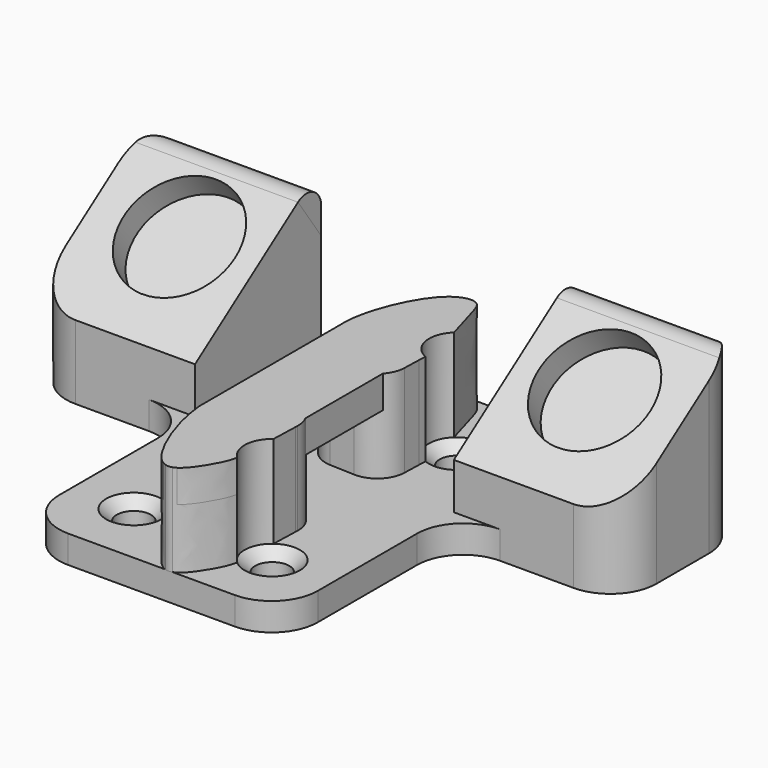
from build123d import *

# Parameters (mm, degrees)
F0_W            = 28.0605573207
F0_H            = 17.1019586477
F1_DEPTH        = 3
F3_DEPTH        = 32
F3_DEPTH_BACK   = 32
F4_DEPTH        = 25
F5_W            = 28.0605573207
F5_H            = 17.0454510609
F5_H_2          = 8.3564384666
F6_REACH        = 49.2047839512
F5_R            = 6.05
F7_DEPTH        = 3
F9_DEPTH        = 10
F10_D           = 3.7
F10_CSINK_D     = 6
F10_CSINK_ANGLE = 90
F12_DEPTH       = 25
F13_DEPTH       = 25
F14_DEPTH       = 5


# Not quite as in the source:
# - a feature names something its author has since deleted; it is built from what else it names


with BuildPart() as f1:
    # F0 (on Top) → F1 (new body)
    with BuildSketch(Plane.XY):
        with BuildLine():
            Line((-19.0302786604, -1.7378998397), (-14.0302786604, -1.7378998397))
            Line((-14.0302786604, -1.7378998397), (-14.0302786604, 15.3640588081))
            Line((-14.0302786604, 15.3640588081), (-27, 15.3640588081))
            ThreePointArc((-27, 15.3640588081), (-30.5355339059, 13.899592714), (-32, 10.3640588081))
            Line((-32, 10.3640588081), (-32, 3.2621001603))
            ThreePointArc((-32, 3.2621001603), (-30.5355339059, -0.2734337456), (-27, -1.7378998397))
            Line((-27, -1.7378998397), (-20.8602603525, -1.7378998397))
            Line((-20.8602603525, -1.7378998397), (-19.0302786604, -1.7378998397))
        make_face()
        with BuildLine():
            ThreePointArc((-14.0302786604, -20.1735929717), (-12.5658125663, -23.7091268776), (-9.0302786604, -25.1735929717))
            Line((-9.0302786604, -25.1735929717), (9.0302786604, -25.1735929717))
            ThreePointArc((9.0302786604, -25.1735929717), (12.5658125663, -23.7091268776), (14.0302786604, -20.1735929717))
            Line((14.0302786604, -20.1735929717), (14.0302786604, -6.7378998397))
            Line((14.0302786604, -6.7378998397), (14.0302786604, -1.7378998397))
            Line((14.0302786604, -1.7378998397), (-14.0302786604, -1.7378998397))
            Line((-14.0302786604, -1.7378998397), (-14.0302786604, -6.7378998397))
            Line((-14.0302786604, -6.7378998397), (-14.0302786604, -20.1735929717))
        make_face()
        with BuildLine():
            Line((14.0302786604, 15.3640588081), (14.0302786604, -1.7378998397))
            Line((14.0302786604, -1.7378998397), (19.0302786604, -1.7378998397))
            Line((19.0302786604, -1.7378998397), (21.6872710735, -1.7378998397))
            Line((21.6872710735, -1.7378998397), (27, -1.7378998397))
            ThreePointArc((27, -1.7378998397), (30.5355339059, -0.2734337456), (32, 3.2621001603))
            Line((32, 3.2621001603), (32, 10.3640588081))
            ThreePointArc((32, 10.3640588081), (30.5355339059, 13.899592714), (27, 15.3640588081))
            Line((27, 15.3640588081), (14.0302786604, 15.3640588081))
        make_face()
        with Locations((0, 6.8130794842)):
            Rectangle(F0_W, F0_H)
        with BuildLine():
            ThreePointArc((-19.0302786604, -1.7378998397), (-15.4947447544, -3.2023659338), (-14.0302786604, -6.7378998397))
            Line((-14.0302786604, -6.7378998397), (-14.0302786604, -1.7378998397))
            Line((-14.0302786604, -1.7378998397), (-19.0302786604, -1.7378998397))
        make_face()
        with BuildLine():
            Line((14.0302786604, -1.7378998397), (14.0302786604, -6.7378998397))
            ThreePointArc((14.0302786604, -6.7378998397), (15.4947447544, -3.2023659338), (19.0302786604, -1.7378998397))
            Line((19.0302786604, -1.7378998397), (14.0302786604, -1.7378998397))
        make_face()
    extrude(amount=F1_DEPTH)

    # F2 (on Right) → F3 (join, two sides)
    with BuildSketch(Plane.YZ) as f3_sk:
        with BuildLine():
            Line((-1.7378998397, 8), (-1.7378998397, 3))
            Line((-1.7378998397, 3), (15.3640588081, 3))
            Line((15.3640588081, 3), (15.3640588081, 16.1534193361))
            ThreePointArc((15.3640588081, 16.1534193361), (14.2866836868, 17.9278948454), (12.2152954749, 17.7905945877))
            Line((12.2152954749, 17.7905945877), (-1.7378998397, 8))
        make_face()
    extrude(amount=F3_DEPTH)
    extrude(f3_sk.sketch, amount=-F3_DEPTH_BACK)

    # F4 (cut): faces of the model
    f4_faces = [f1.faces().sort_by_distance(p)[0] for p in [
        (-30.8831603053, 14.2472191133, 3),
        (-30.8831603053, -0.621060145, 3),
        (30.8831603053, -0.621060145, 3),
        (30.8831603053, 14.2472191133, 3),
    ]]
    extrude(f4_faces, amount=-F4_DEPTH, mode=Mode.SUBTRACT)

    f6_end = Plane(origin=(0, -13.1098018859, 3), x_dir=(1, 0, 0), z_dir=(0, 0, 1))
    # F5 (on face) → F6 (cut, up to a plane its end follows)
    with BuildSketch(Plane(origin=(0, -4.334811805, 6.177814353), x_dir=(1, 0, 0), z_dir=(0, -0.5743816666, 0.8185876258))):
        with Locations((0, 11.6951555593)):
            Rectangle(F5_W, F5_H)
        Polygon((14.0302786604, -5.0207045861), (14.0302786604, 0), (14.0302786604, 3.1724300289), (-14.0302786604, 3.1724300289), (-14.0302786604, 0), (-14.0302786604, -5.0207045861), align=None)
        with Locations((0, 24.396100323)):
            Rectangle(F5_W, F5_H_2)
    f6_long = extrude(amount=-F6_REACH, mode=Mode.PRIVATE)
    add(split(f6_long, bisect_by=f6_end, keep=Keep.TOP, mode=Mode.PRIVATE), mode=Mode.SUBTRACT)

    # F5 (on face) → F7 (cut)
    with BuildSketch(Plane(origin=(0, -4.334811805, 6.177814353), x_dir=(1, 0, 0), z_dir=(0, -0.5743816666, 0.8185876258))):
        with Locations((22.5, 13.5350767523)):
            Circle(F5_R)
        with Locations((-22.5, 13.5350767523)):
            Circle(F5_R)
    extrude(amount=-F7_DEPTH, mode=Mode.SUBTRACT)

    # F8 (on face) → F9 (join)
    with BuildSketch(Plane.XY.offset(3)):
        with BuildLine():
            add(Edge.make_bspline(
                [(3.439653721, 14.4599989291), (4.0052184257, 14.1775319538), (4.2384614527, 13.0214622017), (5.1246291924, 10.2048677906), (5.4504108833, 9.003783584)],
                knots=[0, 0, 0, 0, 0.1106519752, 0.1831613583, 0.1831613583, 0.1831613583, 0.1831613583], degree=3))
            add(Edge.make_bspline(
                [(-2.425625543, 2.1165073176), (-2.6128697036, 2.4416064205), (-3.7900282508, 5.4402549428), (-0.4138105091, 14.2334908767), (2.8259898176, 14.7664886821), (3.439653721, 14.4599989291)],
                knots=[0.6187512381, 0.6187512381, 0.6187512381, 0.6187512381, 0.6507091383, 0.8799374811, 1, 1, 1, 1], degree=3))
            add(Edge.make_bspline(
                [(6.2951599905, 3.2293955823), (6.2536285053, 2.7551424943), (5.7362561971, 0.3058795284), (1.5238317893, -0.5897867433), (-1.6783380052, 0.8190435823), (-2.425625543, 2.1165073176)],
                knots=[0.3006282955, 0.3006282955, 0.3006282955, 0.3006282955, 0.3342495888, 0.491207925, 0.6187512381, 0.6187512381, 0.6187512381, 0.6187512381], degree=3))
            Line((6.2951599905, 3.2293955823), (6.3205224566, 4.054668216))
            ThreePointArc((6.3205224566, 4.054668216), (4.5453166658, 6.2936120697), (5.4504108833, 9.003783584))
        make_face()
        with BuildLine():
            add(Edge.make_bspline(
                [(6.2951599905, 3.2293955823), (6.2536285053, 2.7551424943), (5.7362561971, 0.3058795284), (1.5238317893, -0.5897867433), (-1.6783380052, 0.8190435823), (-2.425625543, 2.1165073176)],
                knots=[0.3006282955, 0.3006282955, 0.3006282955, 0.3006282955, 0.3342495888, 0.491207925, 0.6187512381, 0.6187512381, 0.6187512381, 0.6187512381], degree=3))
            Line((-2.425625543, 2.1165073176), (-2.4419164115, 1.5864165937))
            ThreePointArc((-2.4419164115, 1.5864165937), (-1.6394334925, -0.5495415445), (0.4334442969, -1.5032048363))
            Line((0.4334442969, -1.5032048363), (3.1138092408, -1.6133925553))
            ThreePointArc((3.1138092408, -1.6133925553), (5.2808377949, -0.8120256781), (6.2356171285, 1.2919225271))
            Line((6.2356171285, 1.2919225271), (6.2951599905, 3.2293955823))
        make_face()
        with BuildLine():
            add(Edge.make_bspline(
                [(6.3205224566, 4.054668216), (6.3259320308, 3.7685769845), (6.3182004896, 3.4924978464), (6.2951599905, 3.2293955823)],
                knots=[0.2819761483, 0.2819761483, 0.2819761483, 0.2819761483, 0.3006282955, 0.3006282955, 0.3006282955, 0.3006282955], degree=3))
            Line((6.3205224566, 4.054668216), (6.2951599905, 3.2293955823))
        make_face()
        with BuildLine():
            Line((5.7109985458, -15.7787108495), (5.7995937264, -12.895900563))
            add(Edge.make_bspline(
                [(5.7995937264, -12.895900563), (5.6014543432, -11.957203972), (5.2341196587, -10.747475142), (4.4402012509, -10.0397747357), (4.2548362634, -9.909795659)],
                knots=[0.078280994, 0.078280994, 0.078280994, 0.078280994, 0.1532878364, 0.173703161, 0.173703161, 0.173703161, 0.173703161], degree=3))
            ThreePointArc((4.2548362634, -9.909795659), (3.5782527554, -9.6387470487), (2.8562729835, -9.5388581041))
            Line((2.8562729835, -9.5388581041), (0.2851764489, -9.4984770116))
            add(Edge.make_bspline(
                [(0.2851764489, -9.4984770116), (0.1886962517, -9.5257281074), (-1.4223255568, -10.024145371), (-2.5699293228, -11.1174611467), (-2.8875198131, -12.9131313678)],
                knots=[0.2910251466, 0.2910251466, 0.2910251466, 0.2910251466, 0.2995550952, 0.4354391583, 0.4354391583, 0.4354391583, 0.4354391583], degree=3))
            Line((-2.8875198131, -12.9131313678), (-2.9514315077, -14.9927624413))
            add(Edge.make_bspline(
                [(-2.9514315077, -14.9927624413), (-2.7153775465, -18.0022293403), (-0.7781826645, -23.3457780002), (1.0082290092, -25.0100423947), (1.4971567675, -25.1735929717)],
                knots=[0.4816763185, 0.4816763185, 0.4816763185, 0.4816763185, 0.6642562574, 0.7348765677, 0.7348765677, 0.7348765677, 0.7348765677], degree=3))
            Line((1.4971567675, -25.1735929717), (2.2805444633, -25.1735929717))
            add(Edge.make_bspline(
                [(2.2805444633, -25.1735929717), (3.0961818535, -24.8930551973), (4.5940584593, -22.6765141), (5.2897590721, -21.2040650633), (5.4504108833, -20.3776246156)],
                knots=[0.7729673791, 0.7729673791, 0.7729673791, 0.7729673791, 0.8930756087, 1, 1, 1, 1], degree=3))
            ThreePointArc((5.4504108833, -20.3776246156), (4.5048044555, -18.0172041338), (5.7109985458, -15.7787108495))
        make_face()
        with BuildLine():
            add(Edge.make_bspline(
                [(5.7995937264, -12.895900563), (5.6014543432, -11.957203972), (5.2341196587, -10.747475142), (4.4402012509, -10.0397747357), (4.2548362634, -9.909795659)],
                knots=[0.078280994, 0.078280994, 0.078280994, 0.078280994, 0.1532878364, 0.173703161, 0.173703161, 0.173703161, 0.173703161], degree=3))
            Line((5.7995937264, -12.895900563), (5.8077457332, -12.6306413387))
            ThreePointArc((5.8077457332, -12.6306413387), (5.414657568, -11.0514138893), (4.2548362634, -9.909795659))
        make_face()
        with BuildLine():
            add(Edge.make_bspline(
                [(0.2851764489, -9.4984770116), (0.1886962517, -9.5257281074), (-1.4223255568, -10.024145371), (-2.5699293228, -11.1174611467), (-2.8875198131, -12.9131313678)],
                knots=[0.2910251466, 0.2910251466, 0.2910251466, 0.2910251466, 0.2995550952, 0.4354391583, 0.4354391583, 0.4354391583, 0.4354391583], degree=3))
            Line((0.2851764489, -9.4984770116), (0.173816477, -9.4967280157))
            ThreePointArc((0.173816477, -9.4967280157), (-1.9448049821, -10.32637036), (-2.8718793694, -12.4042049027))
            Line((-2.8718793694, -12.4042049027), (-2.8875198131, -12.9131313678))
        make_face()
        with BuildLine():
            add(Edge.make_bspline(
                [(1.4971567675, -25.1735929717), (1.7608720486, -25.2618080212), (2.0218753444, -25.2625619913), (2.2805444633, -25.1735929717)],
                knots=[0.7348765677, 0.7348765677, 0.7348765677, 0.7348765677, 0.7729673791, 0.7729673791, 0.7729673791, 0.7729673791], degree=3))
            Line((2.2805444633, -25.1735929717), (1.4971567675, -25.1735929717))
        make_face()
    extrude(amount=F9_DEPTH)

    # F10 (through all)
    with Locations(Plane.XY.offset(3)):
        with Locations((-7.5, 6.8130794842), (-7.5, -18.1869205158), (7.5, 6.8130794842), (7.5, -18.1869205158)):
            CounterSinkHole(F10_D / 2, F10_CSINK_D / 2, counter_sink_angle=F10_CSINK_ANGLE)

    # F11 (on Front) → F12 (join)
    with BuildSketch(Plane.XZ):
        with BuildLine():
            Line((-2.9514315077, 9.5), (5.4504108833, 9.5))
            Line((5.4504108833, 9.5), (5.4504108833, 13))
            add(Edge.make_bspline(
                [(5.4504108833, 13), (2.649796753, 13), (-0.1508173774, 13), (-2.9514315077, 13)],
                knots=[0.0010524799, 0.0010524799, 0.0010524799, 0.0010524799, 0.9996431059, 0.9996431059, 0.9996431059, 0.9996431059], degree=3))
            Line((-2.9514315077, 13), (-2.9514315077, 9.5))
        make_face()
    extrude(amount=F12_DEPTH)

    # F13 (cut): faces of the model
    f13_faces = [f1.faces().sort_by_distance(p)[0] for p in [
        (-1.8145257216, -22.2530122303, 9.5),
        (4.6195780711, -23.6613899314, 9.5),
        (5.0645605364, -18.1869205158, 9.5),
        (4.6195780711, -23.6613899314, 9.5),
    ]]
    extrude(f13_faces, amount=-F13_DEPTH, mode=Mode.SUBTRACT)

    # F14 (add): a face of the model
    f14_faces = [f1.faces().sort_by_distance(p)[0] for p in [
        (-2.4980717075, 0, 11.25),
    ]]
    extrude(f14_faces, amount=F14_DEPTH)


solid = f1.part
